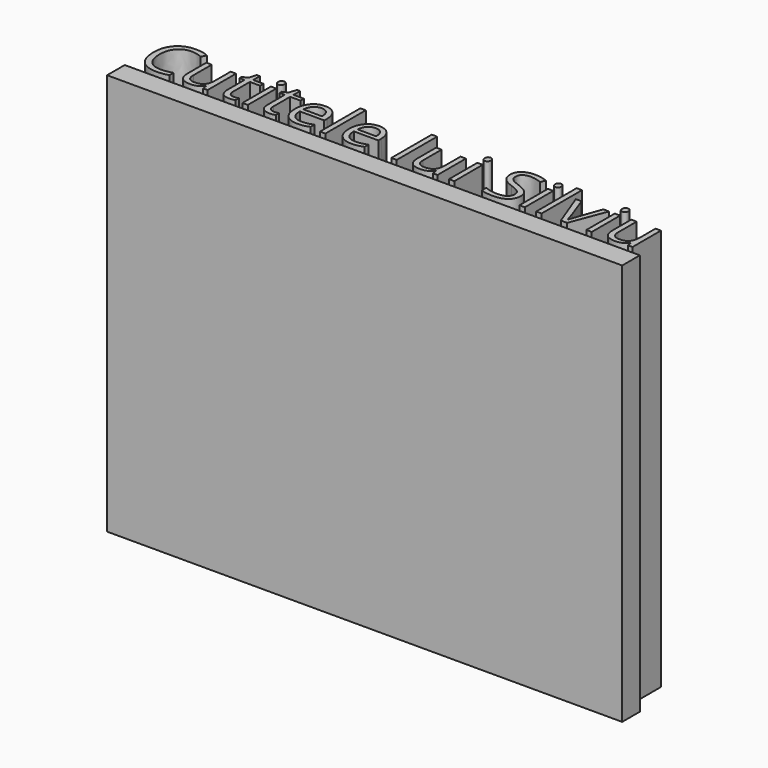
from build123d import *

# Parameters (mm, degrees)
F0_TEXT_SIZE = 8.2667140911
F1_DEPTH     = 50
F2_W         = 64.0988396481
F2_H         = 2.747092396
F3_DEPTH     = 50


# Not quite as in the source:
# - Text() gives the source's letters only with a copy of the font that has no kerning and outlines rounded to 1/6400 em; it was checked with that copy


with BuildPart() as f1:
    # F0 (on Top) → F1 (new body)
    with BuildSketch(Plane.XY):
        with Locations((-70.0508654118, 55.3997084498)):
            Text('Cutitele lui Silviu', F0_TEXT_SIZE, font='Open Sans', text_align=(TextAlign.LEFT, TextAlign.BOTTOM))
    extrude(amount=F1_DEPTH)


with BuildPart() as f3:
    # F2 (on Top) → F3 (new body)
    with BuildSketch(Plane.XY):
        with Locations((-38.0014530383, 53.11046727)):
            Rectangle(F2_W, F2_H)
    extrude(amount=F3_DEPTH)


solid = Compound([f1.part, f3.part])
